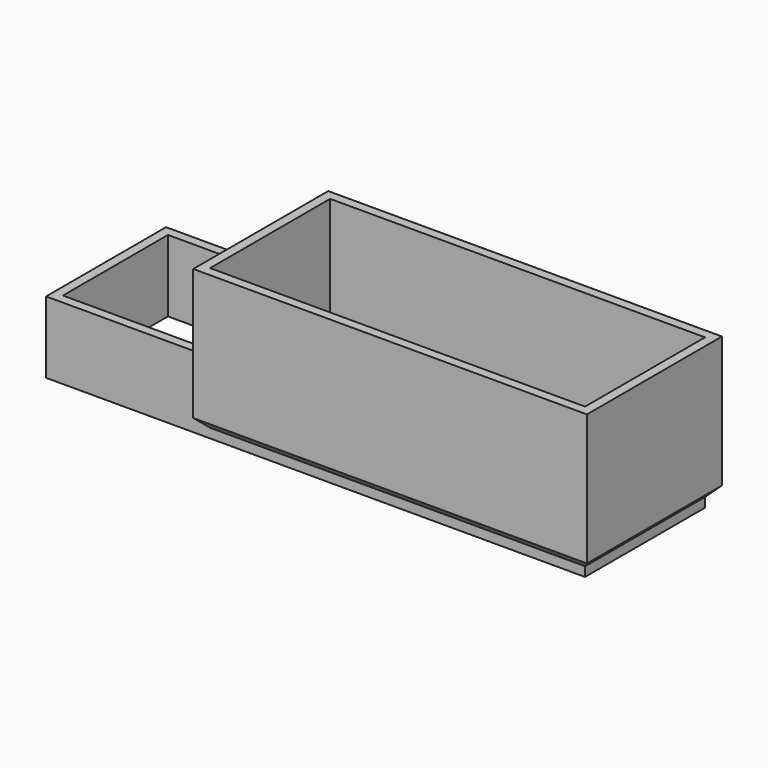
from build123d import *

# Parameters (mm, degrees)
F0_W     = 84
F0_H     = 36
F0_W_2   = 80
F0_H_2   = 32
F1_DEPTH = 30
F0_W_3   = 76
F0_H_3   = 28
F2_DEPTH = 3
F0_R     = 11
F3_DEPTH = 2
F4_SIZE  = 1.99999
F5_SIZE  = 1.99999
F6_W     = 27
F6_H     = 1.99999
F7_DEPTH = 5
F9_DEPTH = 15.3
F10_R    = 0.99999


# Not quite as in the source:
# - a fillet or chamfer is up to 0.001 mm smaller than in the source, because OpenCascade refuses the exact size


with BuildPart() as f1:
    # F0 (on Top) → F1 (new body)
    with BuildSketch(Plane.XY):
        Rectangle(F0_W, F0_H)
        Rectangle(F0_W_2, F0_H_2, mode=Mode.SUBTRACT)
    extrude(amount=F1_DEPTH)

    # F0 (on Top) → F2 (join)
    with BuildSketch(Plane.XY):
        Rectangle(F0_W_2, F0_H_2)
        Rectangle(F0_W_3, F0_H_3, mode=Mode.SUBTRACT)
    extrude(amount=F2_DEPTH)

    # F0 (on Top) → F3 (join)
    with BuildSketch(Plane.XY):
        Rectangle(F0_W_2, F0_H_2)
        Rectangle(F0_W_3, F0_H_3, mode=Mode.SUBTRACT)
        Rectangle(F0_W_3, F0_H_3)
        with Locations((-24.4961753488, 0)):
            Circle(F0_R, mode=Mode.SUBTRACT)
    extrude(amount=-F3_DEPTH)

    # F4 (size 2 in the source; OpenCascade refuses exactly that, so slightly less here)
    f4_edges = [f1.edges().sort_by_distance(p)[0] for p in [
        (0, 18, 0),
        (0, -18, 0),
        (42, 0, 0),
        (-42, 0, 0),
    ]]
    chamfer(f4_edges, length=F4_SIZE)

    # F5 (size 2 in the source; OpenCascade refuses exactly that, so slightly less here)
    f5_edges = [f1.edges().sort_by_distance(p)[0] for p in [
        (0, -14, 3),
        (38, 0, 3),
        (0, 14, 3),
        (-38, 0, 3),
    ]]
    chamfer(f5_edges, length=F5_SIZE)

    # F6 (on face) → F7 (cut)
    with BuildSketch(Plane(origin=(-42, 0, 0), x_dir=(0, -1, 0), z_dir=(-1, 0, 0))):
        with Locations((0, 0.999995)):
            Rectangle(F6_W, F6_H)
    extrude(amount=-F7_DEPTH, mode=Mode.SUBTRACT)

    # F8 (on face) → F9 (join)
    with BuildSketch(Plane(origin=(0, 0, -2), x_dir=(1, 0, 0), z_dir=(0, 0, -1))):
        Polygon((-40, 14), (-40, 16), (-75, 16), (-75, -16), (-40, -16), (-40, -14), (-73, -14), (-73, 14), align=None)
    extrude(amount=-F9_DEPTH)

    # F10 (radius 1 in the source; OpenCascade refuses exactly that, so slightly less here)
    f10_edges = [f1.edges().sort_by_distance(p)[0] for p in [
        (-35.496175, 0, -2),
        (-35.496175, 0, 0),
    ]]
    fillet(f10_edges, radius=F10_R)


solid = f1.part
